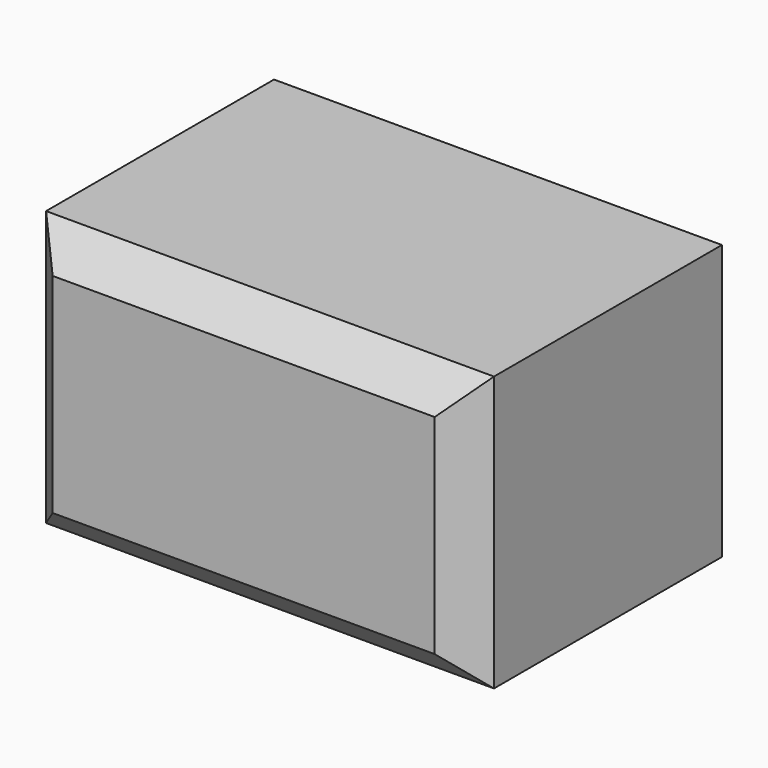
from build123d import *

# Parameters (mm, degrees)
F0_W     = 41.4270346519
F0_H     = 32.4484184384
F1_DEPTH = 25.4
F4_SIZE  = 3.048


# Not quite as in the source:
# - the program builds the solid bodies; features that only make, move or delete a surface that nothing else refers to are left out


with BuildPart() as f1:
    # F0 (on Top) → F1 (new body)
    with BuildSketch(Plane.XY):
        with Locations((-16.9389118673, 7.4230190367)):
            Rectangle(F0_W, F0_H)
    extrude(amount=F1_DEPTH)

    # F4
    f4_edges = [f1.edges().sort_by_distance(p)[0] for p in [
        (3.774605, 23.647228, 12.7),
        (-37.652429, 23.647228, 12.7),
        (-16.938912, 23.647228, 0),
        (-16.938912, 23.647228, 25.4),
        (-37.652429, -8.80119, 12.7),
        (3.774605, -8.80119, 12.7),
        (-16.938912, -8.80119, 0),
        (-16.938912, -8.80119, 25.4),
    ]]
    chamfer(f4_edges, length=F4_SIZE)


solid = f1.part
